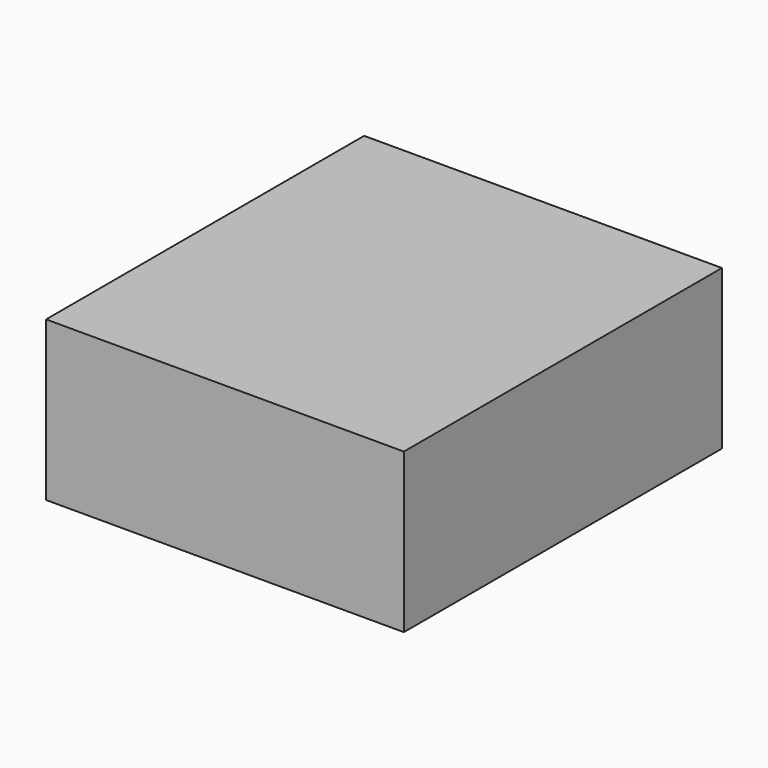
from build123d import *

# Parameters (mm, degrees)
F0_W     = 90
F0_H     = 40
F1_DEPTH = 100


# Not quite as in the source:
# - a feature names something its author has since deleted; it is built from what else it names


with BuildPart() as f1:
    # F0 (on Front) → F1 (new body)
    with BuildSketch(Plane.XZ):
        Rectangle(F0_W, F0_H)
    extrude(amount=F1_DEPTH)


solid = f1.part
